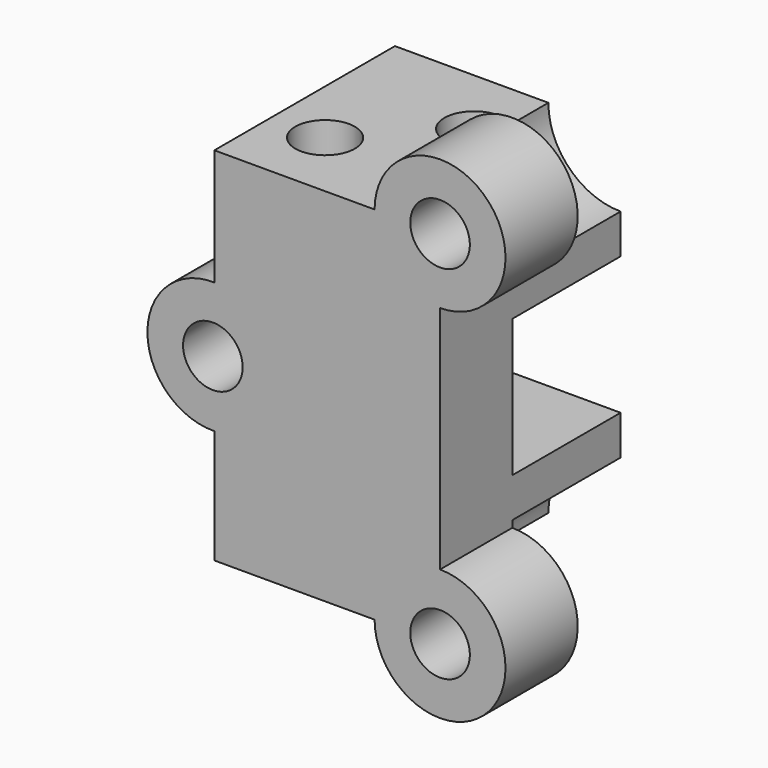
from build123d import *

# Parameters (mm, degrees)
F1_DEPTH       = 25
F3_D           = 13.2
F3_CBORE_D     = 19.25
F3_CBORE_DEPTH = 0
F5_D           = 13.2
F5_CBORE_D     = 19.25
F5_CBORE_DEPTH = 0
F6_W           = 40
F6_H           = 30.5
F7_DEPTH       = 30
F8_R           = 16
F9_DEPTH       = 30.5
F10_R          = 16
F11_DEPTH      = 30


with BuildPart() as f1:
    # F0 (on Front) → F1 (new body, symmetric)
    with BuildSketch(Plane.XZ):
        with BuildLine():
            Line((25, -25.5), (25, -40))
            Line((25, -40), (10.5, -40))
            ThreePointArc((10.5, -40), (25, -54.5), (39.5, -40))
            ThreePointArc((39.5, -40), (35.2530483272, -29.7469516728), (25, -25.5))
        make_face()
        with BuildLine():
            Line((10.5, -40), (25, -40))
            Line((25, -40), (25, -25.5))
            ThreePointArc((25, -25.5), (14.7469516728, -29.7469516728), (10.5, -40))
        make_face()
        with BuildLine():
            Line((-25, -40), (10.5, -40))
            ThreePointArc((10.5, -40), (14.7469516728, -29.7469516728), (25, -25.5))
            Line((25, -25.5), (25, 25.5))
            ThreePointArc((25, 25.5), (14.7469516728, 29.7469516728), (10.5, 40))
            Line((10.5, 40), (-25, 40))
            Line((-25, 40), (-25, 14.2162181315))
            ThreePointArc((-25, 14.2162181315), (-14.9640357801, 9.8540823977), (-10.8347666082, -0.279916916))
            ThreePointArc((-10.8347666082, -0.279916916), (-14.9640357801, -10.4139162298), (-25, -14.7760519636))
            Line((-25, -14.7760519636), (-25, -40))
        make_face()
        with BuildLine():
            ThreePointArc((10.5, 40), (14.7469516728, 29.7469516728), (25, 25.5))
            Line((25, 25.5), (25, 40))
            Line((25, 40), (10.5, 40))
        make_face()
        with BuildLine():
            Line((25, 40), (25, 25.5))
            ThreePointArc((25, 25.5), (35.2530483272, 29.7469516728), (39.5, 40))
            ThreePointArc((39.5, 40), (25, 54.5), (10.5, 40))
            Line((10.5, 40), (25, 40))
        make_face()
        with BuildLine():
            ThreePointArc((-25, 14.2162181315), (-39.8347666082, -0.279916916), (-25, -14.7760519636))
            Line((-25, -14.7760519636), (-25, 14.2162181315))
        make_face()
        with BuildLine():
            Line((-25, 14.2162181315), (-25, -14.7760519636))
            ThreePointArc((-25, -14.7760519636), (-14.9640357801, -10.4139162298), (-10.8347666082, -0.279916916))
            ThreePointArc((-10.8347666082, -0.279916916), (-14.9640357801, 9.8540823977), (-25, 14.2162181315))
        make_face()
    extrude(amount=F1_DEPTH, both=True)

    # F3 (through all)
    with Locations(Plane.XZ.offset(25)):
        with Locations((25, 40), (-25.3347666082, -0.279916916), (25, -40)):
            CounterBoreHole(F3_D / 2, F3_CBORE_D / 2, F3_CBORE_DEPTH)

    # F5 (through all)
    with Locations(Plane.XY.offset(40)):
        with Locations((-13, -9.3407420599), (5.0832007976, 9.3407420599)):
            CounterBoreHole(F5_D / 2, F5_CBORE_D / 2, F5_CBORE_DEPTH)

    # F6 (on face) → F7 (cut)
    with BuildSketch(Plane(origin=(0, 25, 0), x_dir=(-1, 0, 0), z_dir=(0, 1, 0))):
        with Locations((-9.9, 0)):
            Rectangle(F6_W, F6_H)
    extrude(amount=-F7_DEPTH, mode=Mode.SUBTRACT)

    # F8 (on face) → F9 (cut)
    with BuildSketch(Plane.XY.offset(-15.25)):
        with Locations((5.0832007976, 9.3407420599)):
            Circle(F8_R)
    extrude(amount=F9_DEPTH, mode=Mode.SUBTRACT)

    # F10 (on face) → F11 (cut)
    with BuildSketch(Plane(origin=(0, 25, 0), x_dir=(-1, 0, 0), z_dir=(0, 1, 0))):
        with Locations((-25, 40)):
            Circle(F10_R)
        with Locations((-25, -40)):
            Circle(F10_R)
    extrude(amount=-F11_DEPTH, mode=Mode.SUBTRACT)


solid = f1.part
